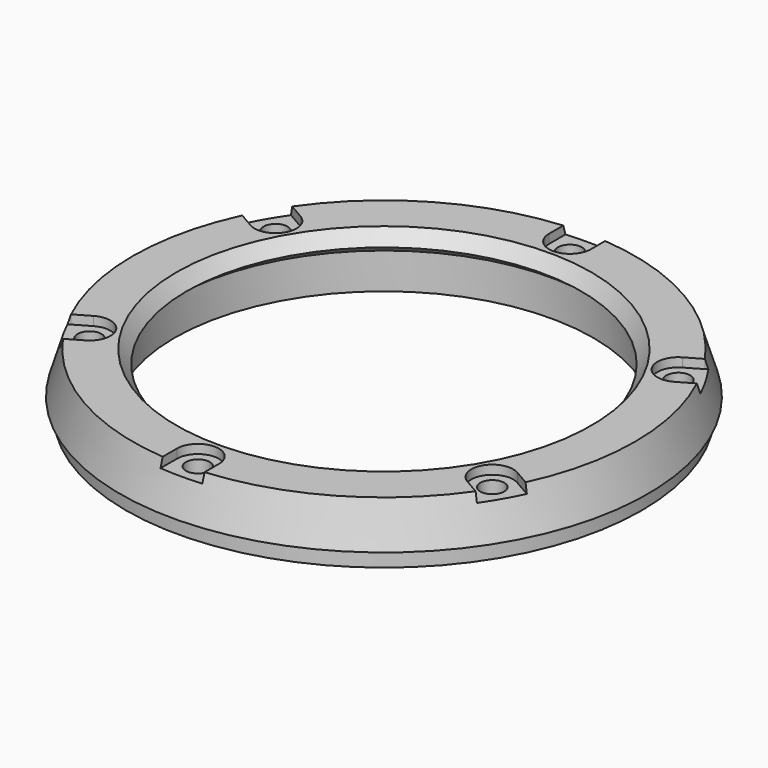
from build123d import *

# Parameters (mm, degrees)
F2_R     = 0.8
F3_DEPTH = 3.901
F4_DEPTH = 0.6
F6_DEPTH = 1.5


with BuildPart() as f1:
    # F0 (on Front) → F1 (revolve)
    with BuildSketch(Plane.XZ):
        Polygon((-14.7, 0), (-14, 0), (-14, 2.4), (-13.2, 3), (-13.875, 3.9), (-16.8, 3.9), (-17.65, 1.1), (-17.25, 1.1), (-17.25, 0), (-16, 0), (-16, 1.5), (-14.7, 1.5), align=None)
    revolve(axis=Axis((0, 0, 5.7374605552), (0, 0, 1)))

    # F2 (on face) → F3 (cut, through all)
    with BuildSketch(Plane.XY.offset(3.9)):
        with Locations((0, 15.55)):
            Circle(F2_R)
        with Locations((13.4666950288, 7.775)):
            Circle(F2_R)
        with Locations((13.4666950288, -7.775)):
            Circle(F2_R)
        with Locations((-13.4666950288, 7.775)):
            Circle(F2_R)
        with Locations((0, -15.55)):
            Circle(F2_R)
        with Locations((-13.4666950288, -7.775)):
            Circle(F2_R)
    extrude(amount=-F3_DEPTH, mode=Mode.SUBTRACT)

    # F2 (on face) → F4 (cut)
    with BuildSketch(Plane.XY.offset(3.9)):
        with BuildLine():
            ThreePointArc((-0.655202269, 16.7872186495), (-1.1994338616, 16.2720515298), (-1.4, 15.55))
            ThreePointArc((-1.4, 15.55), (0, 14.15), (1.4, 15.55))
            ThreePointArc((1.4, 15.55), (1.1994338616, 16.2720515298), (0.655202269, 16.7872186495))
            ThreePointArc((0.655202269, 16.7872186495), (0, 16.8), (-0.655202269, 16.7872186495))
        make_face()
        with Locations((0, 15.55)):
            Circle(F2_R, mode=Mode.SUBTRACT)
        with BuildLine():
            ThreePointArc((0.655202269, 16.7872186495), (1.1994338616, 16.2720515298), (1.4, 15.55))
            Line((1.4, 15.55), (1.4, 16.7415650403))
            ThreePointArc((1.4, 16.7415650403), (1.0278546369, 16.7685275098), (0.655202269, 16.7872186495))
        make_face()
        with BuildLine():
            ThreePointArc((-1.4, 16.7415650403), (-1.0278546369, 16.7685275098), (-0.655202269, 16.7872186495))
            ThreePointArc((-0.655202269, 16.7872186495), (0, 16.95), (0.655202269, 16.7872186495))
            ThreePointArc((0.655202269, 16.7872186495), (1.0278546369, 16.7685275098), (1.4, 16.7415650403))
            Line((1.4, 16.7415650403), (1.4, 17.5943883099))
            ThreePointArc((1.4, 17.5943883099), (0, 17.65), (-1.4, 17.5943883099))
            Line((-1.4, 17.5943883099), (-1.4, 16.7415650403))
        make_face()
        with BuildLine():
            Line((-1.4, 16.7415650403), (-1.4, 15.55))
            ThreePointArc((-1.4, 15.55), (-1.1994338616, 16.2720515298), (-0.655202269, 16.7872186495))
            ThreePointArc((-0.655202269, 16.7872186495), (-1.0278546369, 16.7685275098), (-1.4, 16.7415650403))
        make_face()
        with BuildLine():
            ThreePointArc((14.2105566749, 8.9610311343), (13.4922930657, 9.1747659592), (12.7666950288, 8.9874355653))
            ThreePointArc((12.7666950288, 8.9874355653), (12.2542594635, 7.075), (14.1666950288, 6.5625644347))
            ThreePointArc((14.1666950288, 6.5625644347), (14.6791305941, 7.075), (14.8666950288, 7.775))
            ThreePointArc((14.8666950288, 7.775), (14.866460988, 7.8005980369), (14.8657589439, 7.8261875152))
            ThreePointArc((14.8657589439, 7.8261875152), (14.5492267836, 8.4), (14.2105566749, 8.9610311343))
        make_face()
        with Locations((13.4666950288, 7.775)):
            Circle(F2_R, mode=Mode.SUBTRACT)
        with BuildLine():
            ThreePointArc((14.2105566749, 8.9610311343), (14.008043489, 9.2744119818), (13.798620624, 9.5832180855))
            Line((13.798620624, 9.5832180855), (12.7666950288, 8.9874355653))
            ThreePointArc((12.7666950288, 8.9874355653), (13.4922930657, 9.1747659592), (14.2105566749, 8.9610311343))
        make_face()
        with BuildLine():
            ThreePointArc((14.8666950288, 7.775), (14.6791305941, 7.075), (14.1666950288, 6.5625644347))
            Line((14.1666950288, 6.5625644347), (15.198620624, 7.1583469549))
            ThreePointArc((15.198620624, 7.1583469549), (15.035898126, 7.4941155279), (14.8657589439, 7.8261875152))
            ThreePointArc((14.8657589439, 7.8261875152), (14.866460988, 7.8005980369), (14.8666950288, 7.775))
        make_face()
        with BuildLine():
            Line((14.5371872404, 10.0096297203), (13.798620624, 9.5832180855))
            ThreePointArc((13.798620624, 9.5832180855), (14.008043489, 9.2744119818), (14.2105566749, 8.9610311343))
            ThreePointArc((14.2105566749, 8.9610311343), (14.6791305941, 8.475), (14.8657589439, 7.8261875152))
            ThreePointArc((14.8657589439, 7.8261875152), (15.035898126, 7.4941155279), (15.198620624, 7.1583469549))
            Line((15.198620624, 7.1583469549), (15.9371872404, 7.5847585897))
            ThreePointArc((15.9371872404, 7.5847585897), (15.2853483768, 8.825), (14.5371872404, 10.0096297203))
        make_face()
        with BuildLine():
            ThreePointArc((14.8657589439, -7.8261875152), (15.035898126, -7.4941155279), (15.198620624, -7.1583469549))
            Line((15.198620624, -7.1583469549), (14.1666950288, -6.5625644347))
            ThreePointArc((14.1666950288, -6.5625644347), (14.6791305941, -7.075), (14.8666950288, -7.775))
            ThreePointArc((14.8666950288, -7.775), (14.866460988, -7.8005980369), (14.8657589439, -7.8261875152))
        make_face()
        with BuildLine():
            ThreePointArc((14.8666950288, -7.775), (14.6791305941, -7.075), (14.1666950288, -6.5625644347))
            ThreePointArc((14.1666950288, -6.5625644347), (12.2542594635, -7.075), (12.7666950288, -8.9874355653))
            ThreePointArc((12.7666950288, -8.9874355653), (13.4922930657, -9.1747659592), (14.2105566749, -8.9610311343))
            ThreePointArc((14.2105566749, -8.9610311343), (14.5492267836, -8.4), (14.8657589439, -7.8261875152))
            ThreePointArc((14.8657589439, -7.8261875152), (14.866460988, -7.8005980369), (14.8666950288, -7.775))
        make_face()
        with Locations((13.4666950288, -7.775)):
            Circle(F2_R, mode=Mode.SUBTRACT)
        with BuildLine():
            Line((12.7666950288, -8.9874355653), (13.798620624, -9.5832180855))
            ThreePointArc((13.798620624, -9.5832180855), (14.008043489, -9.2744119818), (14.2105566749, -8.9610311343))
            ThreePointArc((14.2105566749, -8.9610311343), (13.4922930657, -9.1747659592), (12.7666950288, -8.9874355653))
        make_face()
        with BuildLine():
            ThreePointArc((14.2105566749, -8.9610311343), (14.6791305941, -8.475), (14.8657589439, -7.8261875152))
            ThreePointArc((14.8657589439, -7.8261875152), (14.5492267836, -8.4), (14.2105566749, -8.9610311343))
        make_face()
        with BuildLine():
            ThreePointArc((14.5371872404, -10.0096297203), (15.2853483768, -8.825), (15.9371872404, -7.5847585897))
            Line((15.9371872404, -7.5847585897), (15.198620624, -7.1583469549))
            ThreePointArc((15.198620624, -7.1583469549), (15.035898126, -7.4941155279), (14.8657589439, -7.8261875152))
            ThreePointArc((14.8657589439, -7.8261875152), (14.6791305941, -8.475), (14.2105566749, -8.9610311343))
            ThreePointArc((14.2105566749, -8.9610311343), (14.008043489, -9.2744119818), (13.798620624, -9.5832180855))
            Line((13.798620624, -9.5832180855), (14.5371872404, -10.0096297203))
        make_face()
        with BuildLine():
            ThreePointArc((14.8657589439, 7.8261875152), (14.6791305941, 8.475), (14.2105566749, 8.9610311343))
            ThreePointArc((14.2105566749, 8.9610311343), (14.5492267836, 8.4), (14.8657589439, 7.8261875152))
        make_face()
        with BuildLine():
            ThreePointArc((0.655202269, 16.7872186495), (0, 16.95), (-0.655202269, 16.7872186495))
            ThreePointArc((-0.655202269, 16.7872186495), (0, 16.8), (0.655202269, 16.7872186495))
        make_face()
        with BuildLine():
            ThreePointArc((-12.0666950288, 7.775), (-12.2542594635, 8.475), (-12.7666950288, 8.9874355653))
            ThreePointArc((-12.7666950288, 8.9874355653), (-13.4922930657, 9.1747659592), (-14.2105566749, 8.9610311343))
            ThreePointArc((-14.2105566749, 8.9610311343), (-14.5492267836, 8.4), (-14.8657589439, 7.8261875152))
            ThreePointArc((-14.8657589439, 7.8261875152), (-14.6917269273, 7.0972855706), (-14.1666950288, 6.5625644347))
            ThreePointArc((-14.1666950288, 6.5625644347), (-12.7666950288, 6.5625644347), (-12.0666950288, 7.775))
        make_face()
        with Locations((-13.4666950288, 7.775)):
            Circle(F2_R, mode=Mode.SUBTRACT)
        with BuildLine():
            ThreePointArc((-14.2105566749, 8.9610311343), (-14.008043489, 9.2744119818), (-13.798620624, 9.5832180855))
            Line((-13.798620624, 9.5832180855), (-14.5371872404, 10.0096297203))
            ThreePointArc((-14.5371872404, 10.0096297203), (-15.2853483768, 8.825), (-15.9371872404, 7.5847585897))
            Line((-15.9371872404, 7.5847585897), (-15.198620624, 7.1583469549))
            ThreePointArc((-15.198620624, 7.1583469549), (-15.035898126, 7.4941155279), (-14.8657589439, 7.8261875152))
            ThreePointArc((-14.8657589439, 7.8261875152), (-14.6791305941, 8.475), (-14.2105566749, 8.9610311343))
        make_face()
        with BuildLine():
            Line((-12.7666950288, 8.9874355653), (-13.798620624, 9.5832180855))
            ThreePointArc((-13.798620624, 9.5832180855), (-14.008043489, 9.2744119818), (-14.2105566749, 8.9610311343))
            ThreePointArc((-14.2105566749, 8.9610311343), (-13.4922930657, 9.1747659592), (-12.7666950288, 8.9874355653))
        make_face()
        with BuildLine():
            ThreePointArc((-14.1666950288, 6.5625644347), (-14.6917269273, 7.0972855706), (-14.8657589439, 7.8261875152))
            ThreePointArc((-14.8657589439, 7.8261875152), (-15.035898126, 7.4941155279), (-15.198620624, 7.1583469549))
            Line((-15.198620624, 7.1583469549), (-14.1666950288, 6.5625644347))
        make_face()
        with BuildLine():
            ThreePointArc((-12.0666950288, -7.775), (-12.7666950288, -6.5625644347), (-14.1666950288, -6.5625644347))
            ThreePointArc((-14.1666950288, -6.5625644347), (-14.6917269273, -7.0972855706), (-14.8657589439, -7.8261875152))
            ThreePointArc((-14.8657589439, -7.8261875152), (-14.5492267836, -8.4), (-14.2105566749, -8.9610311343))
            ThreePointArc((-14.2105566749, -8.9610311343), (-13.4922930657, -9.1747659592), (-12.7666950288, -8.9874355653))
            ThreePointArc((-12.7666950288, -8.9874355653), (-12.2542594635, -8.475), (-12.0666950288, -7.775))
        make_face()
        with Locations((-13.4666950288, -7.775)):
            Circle(F2_R, mode=Mode.SUBTRACT)
        with BuildLine():
            Line((-14.1666950288, -6.5625644347), (-15.198620624, -7.1583469549))
            ThreePointArc((-15.198620624, -7.1583469549), (-15.035898126, -7.4941155279), (-14.8657589439, -7.8261875152))
            ThreePointArc((-14.8657589439, -7.8261875152), (-14.6917269273, -7.0972855706), (-14.1666950288, -6.5625644347))
        make_face()
        with BuildLine():
            Line((-15.198620624, -7.1583469549), (-15.9371872404, -7.5847585897))
            ThreePointArc((-15.9371872404, -7.5847585897), (-15.2853483768, -8.825), (-14.5371872404, -10.0096297203))
            Line((-14.5371872404, -10.0096297203), (-13.798620624, -9.5832180855))
            ThreePointArc((-13.798620624, -9.5832180855), (-14.008043489, -9.2744119818), (-14.2105566749, -8.9610311343))
            ThreePointArc((-14.2105566749, -8.9610311343), (-14.6791305941, -8.475), (-14.8657589439, -7.8261875152))
            ThreePointArc((-14.8657589439, -7.8261875152), (-15.035898126, -7.4941155279), (-15.198620624, -7.1583469549))
        make_face()
        with BuildLine():
            ThreePointArc((-14.2105566749, -8.9610311343), (-14.5492267836, -8.4), (-14.8657589439, -7.8261875152))
            ThreePointArc((-14.8657589439, -7.8261875152), (-14.6791305941, -8.475), (-14.2105566749, -8.9610311343))
        make_face()
        with BuildLine():
            ThreePointArc((-14.2105566749, -8.9610311343), (-14.008043489, -9.2744119818), (-13.798620624, -9.5832180855))
            Line((-13.798620624, -9.5832180855), (-12.7666950288, -8.9874355653))
            ThreePointArc((-12.7666950288, -8.9874355653), (-13.4922930657, -9.1747659592), (-14.2105566749, -8.9610311343))
        make_face()
        with BuildLine():
            Line((-1.4, -15.55), (-1.4, -16.7415650403))
            ThreePointArc((-1.4, -16.7415650403), (-1.0278546369, -16.7685275098), (-0.655202269, -16.7872186495))
            ThreePointArc((-0.655202269, -16.7872186495), (-1.1994338616, -16.2720515298), (-1.4, -15.55))
        make_face()
        with BuildLine():
            ThreePointArc((0.655202269, -16.7872186495), (1.0278546369, -16.7685275098), (1.4, -16.7415650403))
            Line((1.4, -16.7415650403), (1.4, -15.55))
            ThreePointArc((1.4, -15.55), (1.1994338616, -16.2720515298), (0.655202269, -16.7872186495))
        make_face()
        with BuildLine():
            Line((-1.4, -16.7415650403), (-1.4, -17.5943883099))
            ThreePointArc((-1.4, -17.5943883099), (0, -17.65), (1.4, -17.5943883099))
            Line((1.4, -17.5943883099), (1.4, -16.7415650403))
            ThreePointArc((1.4, -16.7415650403), (1.0278546369, -16.7685275098), (0.655202269, -16.7872186495))
            ThreePointArc((0.655202269, -16.7872186495), (0, -16.95), (-0.655202269, -16.7872186495))
            ThreePointArc((-0.655202269, -16.7872186495), (-1.0278546369, -16.7685275098), (-1.4, -16.7415650403))
        make_face()
        with BuildLine():
            ThreePointArc((0.655202269, -16.7872186495), (0, -16.8), (-0.655202269, -16.7872186495))
            ThreePointArc((-0.655202269, -16.7872186495), (0, -16.95), (0.655202269, -16.7872186495))
        make_face()
        with BuildLine():
            ThreePointArc((1.4, -15.55), (0, -14.15), (-1.4, -15.55))
            ThreePointArc((-1.4, -15.55), (-1.1994338616, -16.2720515298), (-0.655202269, -16.7872186495))
            ThreePointArc((-0.655202269, -16.7872186495), (0, -16.8), (0.655202269, -16.7872186495))
            ThreePointArc((0.655202269, -16.7872186495), (1.1994338616, -16.2720515298), (1.4, -15.55))
        make_face()
        with Locations((0, -15.55)):
            Circle(F2_R, mode=Mode.SUBTRACT)
        with BuildLine():
            ThreePointArc((-14.8657589439, 7.8261875152), (-14.5492267836, 8.4), (-14.2105566749, 8.9610311343))
            ThreePointArc((-14.2105566749, 8.9610311343), (-14.6791305941, 8.475), (-14.8657589439, 7.8261875152))
        make_face()
    extrude(amount=-F4_DEPTH, mode=Mode.SUBTRACT)

    # F5 (on face) → F6 (join, through all)
    with BuildSketch(Plane(origin=(0, 0, 1.5), x_dir=(1, 0, 0), z_dir=(0, 0, -1))):
        with BuildLine():
            ThreePointArc((1.5556276057, -15.9241961415), (1.5888681772, -15.7384089048), (1.6, -15.55))
            ThreePointArc((1.6, -15.55), (1.5275208457, -15.0738906997), (1.3166499177, -14.6409163987))
            ThreePointArc((1.3166499177, -14.6409163987), (0, -14.7), (-1.3166499177, -14.6409163987))
            ThreePointArc((-1.3166499177, -14.6409163987), (-1.5729578086, -15.2570772585), (-1.5556276057, -15.9241961415))
            ThreePointArc((-1.5556276057, -15.9241961415), (-1.113638053, -15.9611970192), (-0.6707927224, -15.9859324759))
            ThreePointArc((-0.6707927224, -15.9859324759), (-0.2273387583, -14.7829816893), (0.8, -15.55))
            ThreePointArc((0.8, -15.55), (0.7670183107, -15.7773387583), (0.6707927224, -15.9859324759))
            ThreePointArc((0.6707927224, -15.9859324759), (1.113638053, -15.9611970192), (1.5556276057, -15.9241961415))
        make_face()
        with BuildLine():
            ThreePointArc((13.3377304948, -6.1802059227), (12.7305734356, -7.35), (12.0210805771, -8.460710476))
            ThreePointArc((12.0210805771, -8.460710476), (12.4265375891, -8.9907600505), (13.0129445905, -9.3093110961))
            ThreePointArc((13.0129445905, -9.3093110961), (13.265983067, -8.9450373542), (13.5088272661, -8.5738897762))
            ThreePointArc((13.5088272661, -8.5738897762), (12.7738747058, -7.375), (14.1796199885, -7.4120426996))
            ThreePointArc((14.1796199885, -7.4120426996), (14.37962112, -7.0161596651), (14.5685721962, -6.6148850454))
            ThreePointArc((14.5685721962, -6.6148850454), (13.9994953976, -6.2663172079), (13.3377304948, -6.1802059227))
        make_face()
        with BuildLine():
            ThreePointArc((-13.0129445905, -9.3093110961), (-12.4265375891, -8.9907600505), (-12.0210805771, -8.460710476))
            ThreePointArc((-12.0210805771, -8.460710476), (-12.7305734356, -7.35), (-13.3377304948, -6.1802059227))
            ThreePointArc((-13.3377304948, -6.1802059227), (-13.9994953976, -6.2663172079), (-14.5685721962, -6.6148850454))
            ThreePointArc((-14.5685721962, -6.6148850454), (-14.37962112, -7.0161596651), (-14.1796199885, -7.4120426996))
            ThreePointArc((-14.1796199885, -7.4120426996), (-13.2800670134, -6.9970732786), (-12.6666950288, -7.775))
            ThreePointArc((-12.6666950288, -7.775), (-12.9161070658, -8.3553902953), (-13.5088272661, -8.5738897762))
            ThreePointArc((-13.5088272661, -8.5738897762), (-13.265983067, -8.9450373542), (-13.0129445905, -9.3093110961))
        make_face()
        with BuildLine():
            ThreePointArc((-14.5685721962, 6.6148850454), (-13.9994953976, 6.2663172079), (-13.3377304948, 6.1802059227))
            ThreePointArc((-13.3377304948, 6.1802059227), (-12.7305734356, 7.35), (-12.0210805771, 8.460710476))
            ThreePointArc((-12.0210805771, 8.460710476), (-12.4265375891, 8.9907600505), (-13.0129445905, 9.3093110961))
            ThreePointArc((-13.0129445905, 9.3093110961), (-13.265983067, 8.9450373542), (-13.5088272661, 8.5738897762))
            ThreePointArc((-13.5088272661, 8.5738897762), (-12.9161070658, 8.3553902953), (-12.6666950288, 7.775))
            ThreePointArc((-12.6666950288, 7.775), (-13.2800670134, 6.9970732786), (-14.1796199885, 7.4120426996))
            ThreePointArc((-14.1796199885, 7.4120426996), (-14.37962112, 7.0161596651), (-14.5685721962, 6.6148850454))
        make_face()
        with BuildLine():
            ThreePointArc((13.3377304948, 6.1802059227), (13.9994953976, 6.2663172079), (14.5685721962, 6.6148850454))
            ThreePointArc((14.5685721962, 6.6148850454), (14.37962112, 7.0161596651), (14.1796199885, 7.4120426996))
            ThreePointArc((14.1796199885, 7.4120426996), (12.7738747058, 7.375), (13.5088272661, 8.5738897762))
            ThreePointArc((13.5088272661, 8.5738897762), (13.265983067, 8.9450373542), (13.0129445905, 9.3093110961))
            ThreePointArc((13.0129445905, 9.3093110961), (12.4265375891, 8.9907600505), (12.0210805771, 8.460710476))
            ThreePointArc((12.0210805771, 8.460710476), (12.7305734356, 7.35), (13.3377304948, 6.1802059227))
        make_face()
        with BuildLine():
            ThreePointArc((-1.5556276057, 15.9241961415), (-1.5729578086, 15.2570772585), (-1.3166499177, 14.6409163987))
            ThreePointArc((-1.3166499177, 14.6409163987), (0, 14.7), (1.3166499177, 14.6409163987))
            ThreePointArc((1.3166499177, 14.6409163987), (1.5275208457, 15.0738906997), (1.6, 15.55))
            ThreePointArc((1.6, 15.55), (1.5888681772, 15.7384089048), (1.5556276057, 15.9241961415))
            ThreePointArc((1.5556276057, 15.9241961415), (1.113638053, 15.9611970192), (0.6707927224, 15.9859324759))
            ThreePointArc((0.6707927224, 15.9859324759), (0.7670183107, 15.7773387583), (0.8, 15.55))
            ThreePointArc((0.8, 15.55), (-0.2273387583, 14.7829816893), (-0.6707927224, 15.9859324759))
            ThreePointArc((-0.6707927224, 15.9859324759), (-1.113638053, 15.9611970192), (-1.5556276057, 15.9241961415))
        make_face()
    extrude(amount=F6_DEPTH)


solid = f1.part
